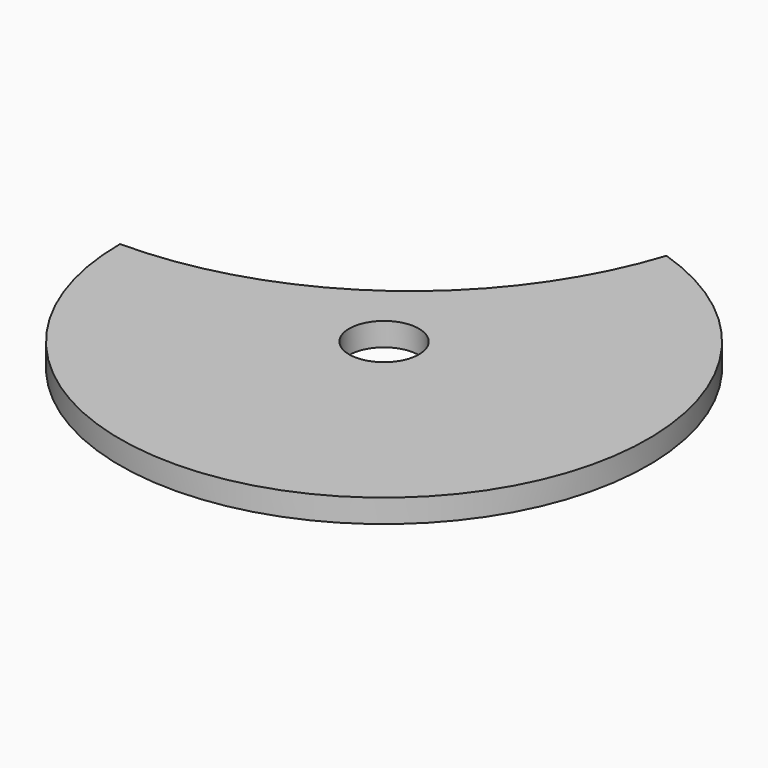
from build123d import *

# Parameters (mm, degrees)
F1_DEPTH = 3.175


# Not quite as in the source:
# - a length typed as a fraction of an inch, garbled in the dataset ("3 / 203.2 mm" for 3/8 in), is restored


with BuildPart() as f1:
    # F0 (on Top) → F1 (new body)
    with BuildSketch(Plane.XY):
        with BuildLine():
            ThreePointArc((-6.8785354807, 9.4567006447), (-20.6864793724, 2.4234489284), (-35.9918, 0))
            ThreePointArc((-35.9918, 0), (21.1544069396, -29.1187351077), (11.1245284011, 34.2294395966))
            ThreePointArc((11.1245284011, 34.2294395966), (4.0851242581, 20.4171352589), (-6.8785354807, 9.4567006447))
        make_face()
        with BuildLine():
            ThreePointArc((4.7625, 0), (0, -4.7625), (-4.7625, 0))
            ThreePointArc((-4.7625, 0), (0, 4.7625), (4.7625, 0))
        make_face(mode=Mode.SUBTRACT)
    extrude(amount=F1_DEPTH)


solid = f1.part
